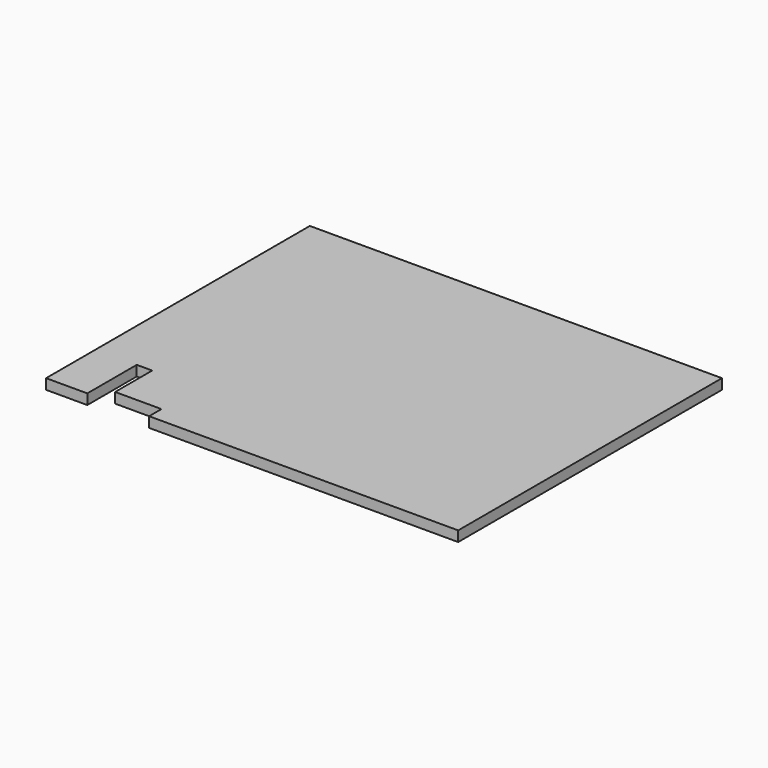
from build123d import *

# Parameters (mm, degrees)
F1_DEPTH = 6.35


# Not quite as in the source:
# - a feature of the source that left no trace in its solid (it failed there, or was rolled back) is left out


with BuildPart() as f1:
    # F0 (on Top) → F1 (new body)
    with BuildSketch(Plane.XY):
        Polygon((127, -101.6), (127, 101.6), (-127, 101.6), (-127, -101.6), (-101.6, -101.6), (-101.6, -63.5), (-92.075, -63.5), (-92.075, -92.075), (-63.5, -92.075), (-63.5, -101.6), align=None)
    extrude(amount=F1_DEPTH)


solid = f1.part
